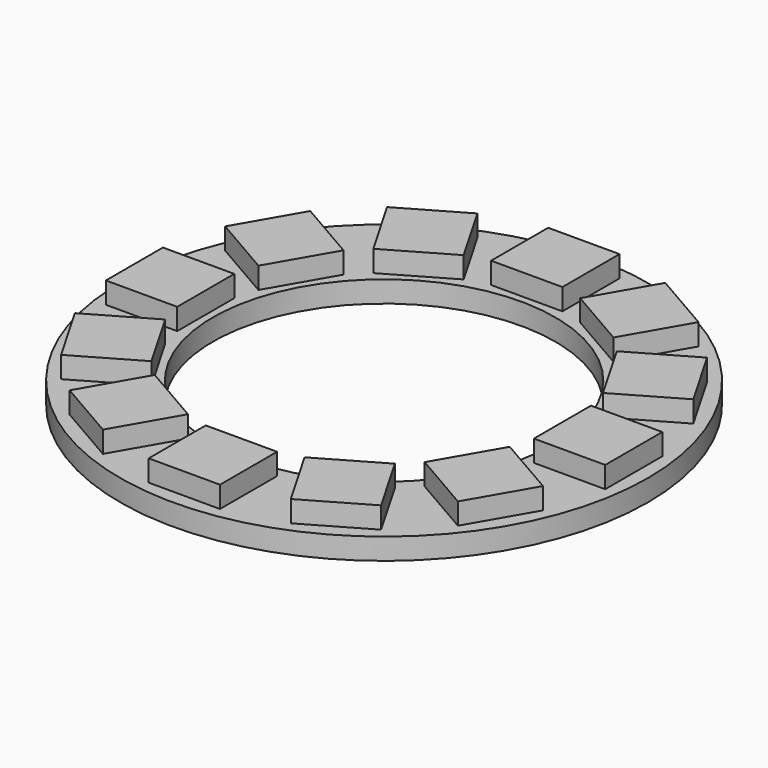
from build123d import *

# Parameters (mm, degrees)
F0_R     = 18.5
F0_R_2   = 12
F1_DEPTH = 1.5
F2_W     = 5
F2_H     = 5
F3_DEPTH = 1.5


# Not quite as in the source:
# - a feature of the source that left no trace in its solid (it failed there, or was rolled back) is left out


with BuildPart() as f1:
    # F0 (on Top) → F1 (new body)
    with BuildSketch(Plane.XY):
        Circle(F0_R)
        Circle(F0_R_2, mode=Mode.SUBTRACT)
    extrude(amount=F1_DEPTH)


with BuildPart() as f3:
    # F2 (on face) → F3 (new body)
    with BuildSketch(Plane.XY.offset(1.5)):
        with Locations((-15, 0)):
            Rectangle(F2_W, F2_H)
    extrude(amount=F3_DEPTH)


with BuildPart() as f3b:
    # F2 (on face) → F3, piece 2 (new body)
    with BuildSketch(Plane.XY.offset(1.5)):
        Polygon((-9.5753175473, -8.4150635095), (-12.0753175473, -4.0849364905), (-16.4054445662, -6.5849364905), (-13.9054445662, -10.9150635095), align=None)
    extrude(amount=F3_DEPTH)


with BuildPart() as f3c:
    # F2 (on face) → F3, piece 3 (new body)
    with BuildSketch(Plane.XY.offset(1.5)):
        Polygon((-4.0849364905, -12.0753175473), (-8.4150635095, -9.5753175473), (-10.9150635095, -13.9054445662), (-6.5849364905, -16.4054445662), align=None)
    extrude(amount=F3_DEPTH)


with BuildPart() as f3d:
    # F2 (on face) → F3, piece 4 (new body)
    with BuildSketch(Plane.XY.offset(1.5)):
        with Locations((0, -15)):
            Rectangle(F2_W, F2_H)
    extrude(amount=F3_DEPTH)


with BuildPart() as f3e:
    # F2 (on face) → F3, piece 5 (new body)
    with BuildSketch(Plane.XY.offset(1.5)):
        Polygon((8.4150635095, -9.5753175473), (4.0849364905, -12.0753175473), (6.5849364905, -16.4054445662), (10.9150635095, -13.9054445662), align=None)
    extrude(amount=F3_DEPTH)


with BuildPart() as f3f:
    # F2 (on face) → F3, piece 6 (new body)
    with BuildSketch(Plane.XY.offset(1.5)):
        Polygon((12.0753175473, -4.0849364905), (9.5753175473, -8.4150635095), (13.9054445662, -10.9150635095), (16.4054445662, -6.5849364905), align=None)
    extrude(amount=F3_DEPTH)


with BuildPart() as f3g:
    # F2 (on face) → F3, piece 7 (new body)
    with BuildSketch(Plane.XY.offset(1.5)):
        with Locations((15, 0)):
            Rectangle(F2_W, F2_H)
    extrude(amount=F3_DEPTH)


with BuildPart() as f3h:
    # F2 (on face) → F3, piece 8 (new body)
    with BuildSketch(Plane.XY.offset(1.5)):
        Polygon((9.5753175473, 8.4150635095), (12.0753175473, 4.0849364905), (16.4054445662, 6.5849364905), (13.9054445662, 10.9150635095), align=None)
    extrude(amount=F3_DEPTH)


with BuildPart() as f3i:
    # F2 (on face) → F3, piece 9 (new body)
    with BuildSketch(Plane.XY.offset(1.5)):
        Polygon((4.0849364905, 12.0753175473), (8.4150635095, 9.5753175473), (10.9150635095, 13.9054445662), (6.5849364905, 16.4054445662), align=None)
    extrude(amount=F3_DEPTH)


with BuildPart() as f3j:
    # F2 (on face) → F3, piece 10 (new body)
    with BuildSketch(Plane.XY.offset(1.5)):
        with Locations((0, 15)):
            Rectangle(F2_W, F2_H)
    extrude(amount=F3_DEPTH)


with BuildPart() as f3k:
    # F2 (on face) → F3, piece 11 (new body)
    with BuildSketch(Plane.XY.offset(1.5)):
        Polygon((-8.4150635095, 9.5753175473), (-4.0849364905, 12.0753175473), (-6.5849364905, 16.4054445662), (-10.9150635095, 13.9054445662), align=None)
    extrude(amount=F3_DEPTH)


with BuildPart() as f3l:
    # F2 (on face) → F3, piece 12 (new body)
    with BuildSketch(Plane.XY.offset(1.5)):
        Polygon((-12.0753175473, 4.0849364905), (-9.5753175473, 8.4150635095), (-13.9054445662, 10.9150635095), (-16.4054445662, 6.5849364905), align=None)
    extrude(amount=F3_DEPTH)


solid = Compound([f1.part, f3.part, f3b.part, f3c.part, f3d.part, f3e.part, f3f.part, f3g.part, f3h.part, f3i.part, f3j.part, f3k.part, f3l.part])
